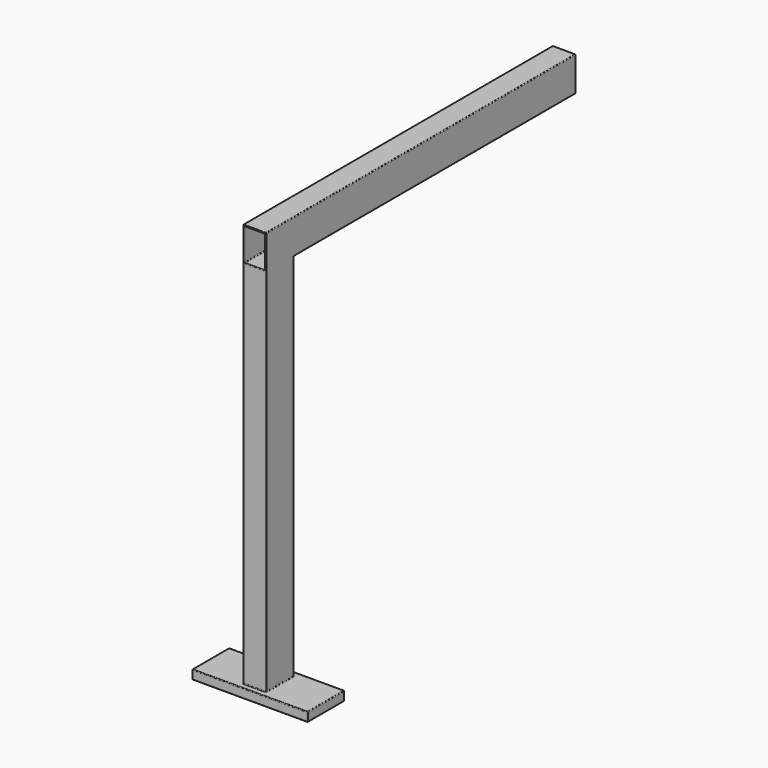
from build123d import *

# Parameters (mm, degrees)
F0_W     = 250
F0_H     = 100
F1_DEPTH = 20
F2_W     = 50
F2_H     = 75
F2_W_2   = 44
F2_H_2   = 69
F3_DEPTH = 800
F4_W     = 50
F4_H     = 75
F4_W_2   = 44
F4_H_2   = 69
F5_DEPTH = 837.2
F6_F1_R  = 1.5
F6_F2_R  = 1.5
F6_F3_R  = 1.5
F6_F4_R  = 1.4999


# Not quite as in the source:
# - a fillet or chamfer is up to 0.001 mm smaller than in the source, because OpenCascade refuses the exact size


with BuildPart() as f1:
    # F0 (on Top) → F1 (new body)
    with BuildSketch(Plane.XY):
        Rectangle(F0_W, F0_H)
    extrude(amount=F1_DEPTH)

    # F2 (on face) → F3 (join)
    with BuildSketch(Plane.XY.offset(20)):
        Rectangle(F2_W, F2_H)
        Rectangle(F2_W_2, F2_H_2, mode=Mode.SUBTRACT)
    extrude(amount=F3_DEPTH)

    # F4 (on face) → F5 (join)
    with BuildSketch(Plane.XZ.offset(37.5)):
        with Locations((0, 857.5)):
            Rectangle(F4_W, F4_H)
        with Locations((0, 857.5)):
            Rectangle(F4_W_2, F4_H_2, mode=Mode.SUBTRACT)
    extrude(amount=-F5_DEPTH)

    # F6: fillet of radius 1.5 on 44 edges, made by hand

    # F6_f1
    f6_f1_edges = [f1.edges().sort_by_distance(p)[0] for p in [
        (-22, -34.5, 420),
        (22, 34.5, 420),
        (22, -34.5, 420),
        (-22, 34.5, 420),
        (-22, 381.1, 892),
        (22, 381.1, 892),
        (0, 37.5, 820),
        (22, 381.1, 823),
        (-22, 381.1, 823),
        (22, 0, 820),
        (0, -34.5, 820),
        (-22, 0, 820),
        (0, 34.5, 820),
        (0, 34.5, 20),
        (-22, 0, 20),
        (22, 0, 20),
        (0, -34.5, 20),
    ]]
    fillet(f6_f1_edges, radius=F6_F1_R)

    # F6_f2
    f6_f2_edges = [f1.edges().sort_by_distance(p)[0] for p in [
        (-25, -37.5, 457.5),
        (25, 37.5, 419.25),
        (25, -37.5, 457.5),
        (-25, 37.5, 419.25),
        (25, 381.1, 895),
        (-25, 381.1, 895),
        (0, -37.5, 895),
        (125, -50, 10),
        (-125, -50, 10),
        (125, 50, 10),
        (0, -50, 0),
        (0, -50, 20),
        (0, 50, 20),
        (125, 0, 20),
        (-125, 0, 20),
        (-125, 50, 10),
        (0, 50, 0),
        (125, 0, 0),
        (-125, 0, 0),
        (-25, 37.9393398282, 819.5606601718),
        (25, 37.9393398282, 819.5606601718),
    ]]
    fillet(f6_f2_edges, radius=F6_F2_R)

    # F6_f3
    f6_f3_edges = [f1.edges().sort_by_distance(p)[0] for p in [
        (25, 0, 20),
        (-25, 0, 20),
        (0, -37.5, 20),
        (0, 37.5, 20),
        (24.5606601718, 37.0606601718, 20),
        (-24.5606601718, 37.0606601718, 20),
        (-24.5606601718, -37.0606601718, 20),
        (24.5606601718, -37.0606601718, 20),
    ]]
    fillet(f6_f3_edges, radius=F6_F3_R)

    # F6_f4 (radius 1.5 in the source; OpenCascade refuses exactly that, so slightly less here)
    f6_f4_edges = [f1.edges().sort_by_distance(p)[0] for p in [
        (-22, -37.5, 857.5),
        (0, -37.5, 823),
        (0, -37.5, 892),
        (22, -37.5, 857.5),
        (21.5606601718, -37.5, 891.5606601718),
        (21.5606601718, -37.5, 823.4393398282),
        (-21.5606601718, -37.5, 891.5606601718),
        (-21.5606601718, -37.5, 823.4393398282),
    ]]
    fillet(f6_f4_edges, radius=F6_F4_R)


solid = f1.part
